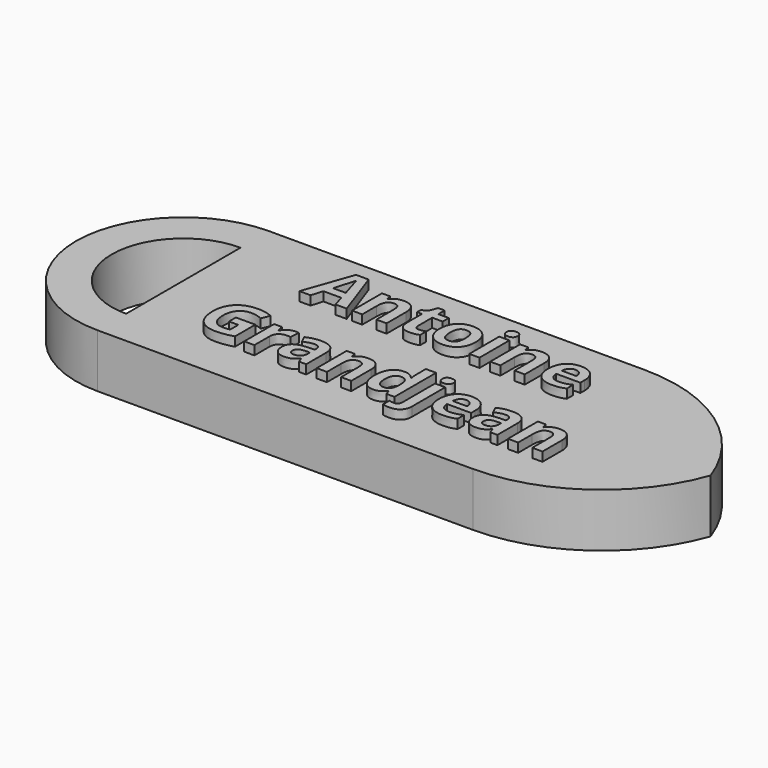
from build123d import *

# Parameters (mm, degrees)
F1_DEPTH     = 3
F2_TEXT_SIZE = 3.8321058619
F3_DEPTH     = 0.508
F4_T1_DEPTH  = 48.0709529959


# Not quite as in the source:
# - a fillet or chamfer that OpenCascade refuses, or shapes differently, is made with other operations: its cross-section is extruded or revolved along the edge and cut away or added
# - Text() gives the source's letters only with a copy of the font that has no kerning and outlines rounded to 1/6400 em; it was checked with that copy


with BuildPart() as f1:
    # F0 (on Top) → F1 (new body)
    with BuildSketch(Plane.XY):
        with BuildLine():
            ThreePointArc((0, 12), (-6, 6), (0, 0))
            Line((0, 0), (0, 2))
            ThreePointArc((0, 2), (-4, 6), (0, 10))
            Line((0, 10), (0, 12))
        make_face()
        with BuildLine():
            Line((0, 2), (0, 0))
            Line((0, 0), (30, 0))
            Line((30, 0), (30, 12))
            Line((30, 12), (0, 12))
            Line((0, 12), (0, 10))
            ThreePointArc((0, 10), (2.8284271247, 8.8284271247), (4, 6))
            ThreePointArc((4, 6), (2.8284271247, 3.1715728753), (0, 2))
        make_face()
        with BuildLine():
            Line((0, 10), (0, 2))
            ThreePointArc((0, 2), (2.8284271247, 3.1715728753), (4, 6))
            ThreePointArc((4, 6), (2.8284271247, 8.8284271247), (0, 10))
        make_face()
    extrude(amount=F1_DEPTH)

    # F2 (on face) → F3 (join)
    with BuildSketch(Plane.XY.offset(3)):
        with Locations((5.1828651725, 7.6336567919)):
            Text('Antoine', F2_TEXT_SIZE, font='Open Sans', font_style=FontStyle.BOLD, text_align=(TextAlign.LEFT, TextAlign.BOTTOM))
        with Locations((3.1913676574, 2.4219928197)):
            Text('Grandjean', F2_TEXT_SIZE, font='Open Sans', font_style=FontStyle.BOLD, text_align=(TextAlign.LEFT, TextAlign.BOTTOM))
    extrude(amount=F3_DEPTH)

    # F4: fillet of radius 9.0141905992 on 2 edges, made by hand

    # F4_s2 → F4_t1 (cut)
    with BuildSketch(Plane.XY.offset(-22.535476498)):
        with BuildLine():
            ThreePointArc((30, 2.9858094008), (27.3598047004, 9.3598047004), (20.9858094008, 12))
            Line((20.9858094008, 12), (30, 12))
            Line((30, 12), (30, 2.9858094008))
        make_face()
        with BuildLine():
            ThreePointArc((20.9858094008, 0), (27.3598047004, 2.6401952996), (30, 9.0141905992))
            Line((30, 9.0141905992), (30, 0))
            Line((30, 0), (20.9858094008, 0))
        make_face()
    extrude(amount=F4_T1_DEPTH, mode=Mode.SUBTRACT)


solid = f1.part
